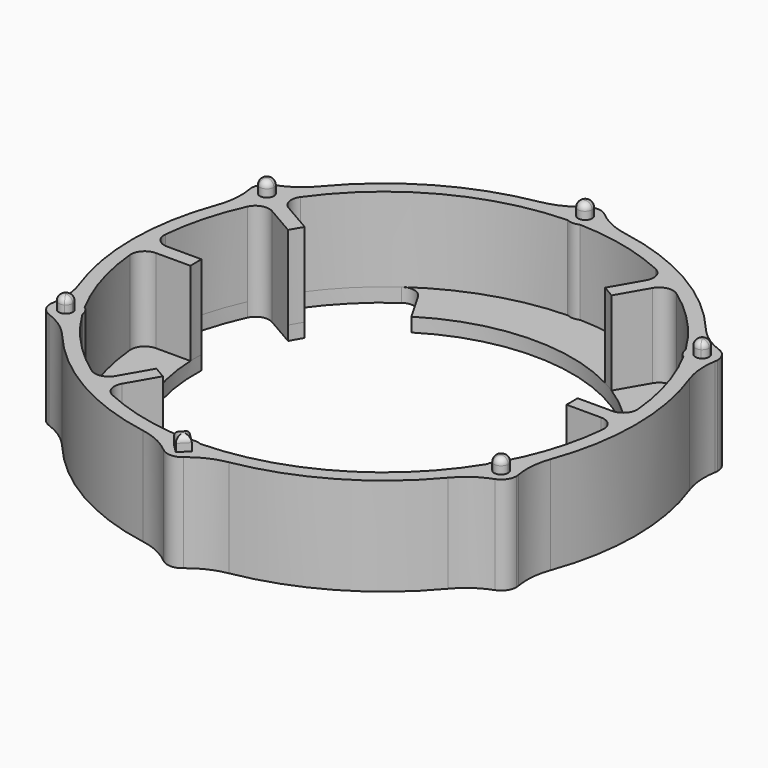
from build123d import *

# Parameters (mm, degrees)
F1_R         = 18
F1_R_2       = 17
F2_DEPTH     = 7
F3_DEPTH     = 7
F4_DEPTH     = 1
F6_DEPTH     = 7
F7_R         = 1
F8_R         = 5
F9_DEPTH     = 8
F10_R        = 0.44999
F11_DEPTH    = 1.8
F12_R        = 13.47
F13_DEPTH    = 1
F14_DEPTH    = 1
F15_T1_DEPTH = 1
F15_T3_DEPTH = 3.7395798703


# Not quite as in the source:
# - a fillet or chamfer that OpenCascade refuses, or shapes differently, is made with other operations: its cross-section is extruded or revolved along the edge and cut away or added
# - a fillet or chamfer is up to 0.001 mm smaller than in the source, because OpenCascade refuses the exact size


with BuildPart() as f2:
    # F1 (on Top) → F2 (new body)
    with BuildSketch(Plane.XY):
        Circle(F1_R)
        Circle(F1_R_2, mode=Mode.SUBTRACT)
    extrude(amount=F2_DEPTH)

    # F0 (on Top) → F3 (join)
    with BuildSketch(Plane.XY):
        with BuildLine():
            Line((-11.4073228059, 7.1633711619), (-14.4660626528, 8.9293354359))
            ThreePointArc((-14.4660626528, 8.9293354359), (-14.7224318643, 8.5), (-14.9660626528, 8.0633100321))
            Line((-14.9660626528, 8.0633100321), (-11.9073228059, 6.2973457581))
            ThreePointArc((-11.9073228059, 6.2973457581), (-11.665362189, 6.735), (-11.4073228059, 7.1633711619))
        make_face()
        with BuildLine():
            Line((7.1633711619, 11.4073228059), (8.9293354359, 14.4660626528))
            ThreePointArc((8.9293354359, 14.4660626528), (8.5, 14.7224318643), (8.0633100321, 14.9660626528))
            Line((8.0633100321, 14.9660626528), (6.2973457581, 11.9073228059))
            ThreePointArc((6.2973457581, 11.9073228059), (6.735, 11.665362189), (7.1633711619, 11.4073228059))
        make_face()
        with BuildLine():
            ThreePointArc((17, 0), (16.9981612676, 0.2500270431), (16.992645468, 0.5))
            Line((16.992645468, 0.5), (13.46071692, 0.5))
            ThreePointArc((13.46071692, 0.5), (13.46767903, 0.2500430841), (13.47, 0))
            ThreePointArc((13.47, 0), (13.46767903, -0.2500430841), (13.46071692, -0.5))
            Line((13.46071692, -0.5), (16.992645468, -0.5))
            ThreePointArc((16.992645468, -0.5), (16.9981612676, -0.2500270431), (17, 0))
        make_face()
        with BuildLine():
            ThreePointArc((-8.9293354359, -14.4660626528), (-8.5, -14.7224318643), (-8.0633100321, -14.9660626528))
            Line((-8.0633100321, -14.9660626528), (-6.2973457581, -11.9073228059))
            ThreePointArc((-6.2973457581, -11.9073228059), (-6.735, -11.665362189), (-7.1633711619, -11.4073228059))
            Line((-7.1633711619, -11.4073228059), (-8.9293354359, -14.4660626528))
        make_face()
        with BuildLine():
            Line((-13.46071692, 0.5), (-16.992645468, 0.5))
            ThreePointArc((-16.992645468, 0.5), (-17, 0), (-16.992645468, -0.5))
            Line((-16.992645468, -0.5), (-13.46071692, -0.5))
            ThreePointArc((-13.46071692, -0.5), (-13.47, 0), (-13.46071692, 0.5))
        make_face()
    extrude(amount=F3_DEPTH)

    # F1 (on Top) → F4 (join)
    with BuildSketch(Plane.XY):
        Circle(F1_R)
        Circle(F1_R_2, mode=Mode.SUBTRACT)
        Circle(F1_R_2)
    extrude(amount=F4_DEPTH)

    # F5 (on Top) → F6 (join)
    with BuildSketch(Plane.XY):
        with BuildLine():
            ThreePointArc((-14.4884572681, 9), (-14.6275367743, 9.5353800561), (-15.0096060035, 9.935377578))
            ThreePointArc((-15.0096060035, 9.935377578), (-15.1731450826, 9.6837837802), (-15.3324673166, 9.4294987133))
            ThreePointArc((-15.3324673166, 9.4294987133), (-15.153718855, 9.2469868663), (-15.0884572681, 9))
            ThreePointArc((-15.0884572681, 9), (-15.3354561915, 8.5687338928), (-15.832419089, 8.5635568422))
            ThreePointArc((-15.832419089, 8.5635568422), (-15.9729752997, 8.2984372068), (-16.1090923805, 8.0310113108))
            ThreePointArc((-16.1090923805, 8.0310113108), (-15.0239657375, 8.0558870238), (-14.4884572681, 9))
        make_face()
        with BuildLine():
            ThreePointArc((-15.3324673166, 9.4294987133), (-15.1731450826, 9.6837837802), (-15.0096060035, 9.935377578))
            ThreePointArc((-15.0096060035, 9.935377578), (-16.5410852123, 9.55), (-16.1090923805, 8.0310113108))
            ThreePointArc((-16.1090923805, 8.0310113108), (-15.9729752997, 8.2984372068), (-15.832419089, 8.5635568422))
            ThreePointArc((-15.832419089, 8.5635568422), (-16.02146997, 9.25), (-15.3324673166, 9.4294987133))
        make_face()
        with BuildLine():
            ThreePointArc((-1.099486377, 17.9663888889), (0, 16.9), (1.099486377, 17.9663888889))
            ThreePointArc((1.099486377, 17.9663888889), (0.7998302171, 17.982220987), (0.4999517724, 17.9930555556))
            ThreePointArc((0.4999517724, 17.9930555556), (0, 17.5), (-0.4999517724, 17.9930555556))
            ThreePointArc((-0.4999517724, 17.9930555556), (-0.7998302171, 17.982220987), (-1.099486377, 17.9663888889))
        make_face()
        with BuildLine():
            ThreePointArc((0.4999517724, 17.9930555556), (0.7998302171, 17.982220987), (1.099486377, 17.9663888889))
            ThreePointArc((1.099486377, 17.9663888889), (1.0998715868, 17.9831924823), (1.1, 18))
            ThreePointArc((1.1, 18), (-0.0168075177, 19.0998715868), (-1.099486377, 17.9663888889))
            ThreePointArc((-1.099486377, 17.9663888889), (-0.7998302171, 17.982220987), (-0.4999517724, 17.9930555556))
            ThreePointArc((-0.4999517724, 17.9930555556), (-0.003472306, 18.4999879429), (0.5, 18))
            ThreePointArc((0.5, 18), (0.4999879429, 17.996527694), (0.4999517724, 17.9930555556))
        make_face()
        with BuildLine():
            ThreePointArc((15.832419089, 8.5635568422), (15.9729752997, 8.2984372068), (16.1090923805, 8.0310113108))
            ThreePointArc((16.1090923805, 8.0310113108), (16.5325702443, 8.4355084694), (16.6884572681, 9))
            ThreePointArc((16.6884572681, 9), (16.1238373242, 9.9609204939), (15.0096060035, 9.935377578))
            ThreePointArc((15.0096060035, 9.935377578), (15.1731450826, 9.6837837802), (15.3324673166, 9.4294987133))
            ThreePointArc((15.3324673166, 9.4294987133), (15.8354441344, 9.4347384132), (16.0884572681, 9))
            ThreePointArc((16.0884572681, 9), (16.0197233753, 8.7469989234), (15.832419089, 8.5635568422))
        make_face()
        with BuildLine():
            ThreePointArc((15.0096060035, 9.935377578), (14.635829324, 8.45), (16.1090923805, 8.0310113108))
            ThreePointArc((16.1090923805, 8.0310113108), (15.9729752997, 8.2984372068), (15.832419089, 8.5635568422))
            ThreePointArc((15.832419089, 8.5635568422), (15.1554445662, 8.75), (15.3324673166, 9.4294987133))
            ThreePointArc((15.3324673166, 9.4294987133), (15.1731450826, 9.6837837802), (15.0096060035, 9.935377578))
        make_face()
        with BuildLine():
            ThreePointArc((-15.3324673166, -9.4294987133), (-15.1731450826, -9.6837837802), (-15.0096060035, -9.935377578))
            ThreePointArc((-15.0096060035, -9.935377578), (-14.6275367743, -9.5353800561), (-14.4884572681, -9))
            ThreePointArc((-14.4884572681, -9), (-15.0239657375, -8.0558870238), (-16.1090923805, -8.0310113108))
            ThreePointArc((-16.1090923805, -8.0310113108), (-15.9729752997, -8.2984372068), (-15.832419089, -8.5635568422))
            ThreePointArc((-15.832419089, -8.5635568422), (-15.3354561915, -8.5687338928), (-15.0884572681, -9))
            ThreePointArc((-15.0884572681, -9), (-15.153718855, -9.2469868663), (-15.3324673166, -9.4294987133))
        make_face()
        with BuildLine():
            ThreePointArc((-16.1090923805, -8.0310113108), (-16.5410852123, -9.55), (-15.0096060035, -9.935377578))
            ThreePointArc((-15.0096060035, -9.935377578), (-15.1731450826, -9.6837837802), (-15.3324673166, -9.4294987133))
            ThreePointArc((-15.3324673166, -9.4294987133), (-16.02146997, -9.25), (-15.832419089, -8.5635568422))
            ThreePointArc((-15.832419089, -8.5635568422), (-15.9729752997, -8.2984372068), (-16.1090923805, -8.0310113108))
        make_face()
        with BuildLine():
            ThreePointArc((0.6255239257, -17.9891278226), (0.8625800837, -17.9793202207), (1.099486377, -17.9663888889))
            ThreePointArc((1.099486377, -17.9663888889), (0, -16.9), (-1.099486377, -17.9663888889))
            ThreePointArc((-1.099486377, -17.9663888889), (-0.8625800837, -17.9793202207), (-0.6255239257, -17.9891278226))
            Line((-0.6255239257, -17.9891278226), (0, -17.3636038969))
            Line((0, -17.3636038969), (0.6255239257, -17.9891278226))
        make_face()
        with BuildLine():
            ThreePointArc((1.1, -18), (1.0998715868, -17.9831924823), (1.099486377, -17.9663888889))
            ThreePointArc((1.099486377, -17.9663888889), (0.8625800837, -17.9793202207), (0.6255239257, -17.9891278226))
            Line((0.6255239257, -17.9891278226), (0.6363961031, -18))
            Line((0.6363961031, -18), (0, -18.6363961031))
            Line((0, -18.6363961031), (-0.6363961031, -18))
            Line((-0.6363961031, -18), (-0.6255239257, -17.9891278226))
            ThreePointArc((-0.6255239257, -17.9891278226), (-0.8625800837, -17.9793202207), (-1.099486377, -17.9663888889))
            ThreePointArc((-1.099486377, -17.9663888889), (-0.0168075177, -19.0998715868), (1.1, -18))
        make_face()
        with BuildLine():
            ThreePointArc((16.6884572681, -9), (16.5325702443, -8.4355084694), (16.1090923805, -8.0310113108))
            ThreePointArc((16.1090923805, -8.0310113108), (15.9729752997, -8.2984372068), (15.832419089, -8.5635568422))
            ThreePointArc((15.832419089, -8.5635568422), (16.0197233753, -8.7469989234), (16.0884572681, -9))
            ThreePointArc((16.0884572681, -9), (15.8354441344, -9.4347384132), (15.3324673166, -9.4294987133))
            ThreePointArc((15.3324673166, -9.4294987133), (15.1731450826, -9.6837837802), (15.0096060035, -9.935377578))
            ThreePointArc((15.0096060035, -9.935377578), (16.1238373242, -9.9609204939), (16.6884572681, -9))
        make_face()
        with BuildLine():
            ThreePointArc((15.832419089, -8.5635568422), (15.9729752997, -8.2984372068), (16.1090923805, -8.0310113108))
            ThreePointArc((16.1090923805, -8.0310113108), (14.635829324, -8.45), (15.0096060035, -9.935377578))
            ThreePointArc((15.0096060035, -9.935377578), (15.1731450826, -9.6837837802), (15.3324673166, -9.4294987133))
            ThreePointArc((15.3324673166, -9.4294987133), (15.1554445662, -8.75), (15.832419089, -8.5635568422))
        make_face()
        with BuildLine():
            ThreePointArc((-15.0884572681, 9), (-15.153718855, 9.2469868663), (-15.3324673166, 9.4294987133))
            ThreePointArc((-15.3324673166, 9.4294987133), (-15.5884572681, 9), (-15.832419089, 8.5635568422))
            ThreePointArc((-15.832419089, 8.5635568422), (-15.3354561915, 8.5687338928), (-15.0884572681, 9))
        make_face()
        with BuildLine():
            ThreePointArc((-15.832419089, 8.5635568422), (-15.5884572681, 9), (-15.3324673166, 9.4294987133))
            ThreePointArc((-15.3324673166, 9.4294987133), (-16.02146997, 9.25), (-15.832419089, 8.5635568422))
        make_face()
        with BuildLine():
            ThreePointArc((-0.4999517724, 17.9930555556), (0, 18), (0.4999517724, 17.9930555556))
            ThreePointArc((0.4999517724, 17.9930555556), (0.4999879429, 17.996527694), (0.5, 18))
            ThreePointArc((0.5, 18), (-0.003472306, 18.4999879429), (-0.4999517724, 17.9930555556))
        make_face()
        with BuildLine():
            ThreePointArc((-0.4999517724, 17.9930555556), (0, 17.5), (0.4999517724, 17.9930555556))
            ThreePointArc((0.4999517724, 17.9930555556), (0, 18), (-0.4999517724, 17.9930555556))
        make_face()
        with BuildLine():
            ThreePointArc((15.3324673166, 9.4294987133), (15.5884572681, 9), (15.832419089, 8.5635568422))
            ThreePointArc((15.832419089, 8.5635568422), (16.0197233753, 8.7469989234), (16.0884572681, 9))
            ThreePointArc((16.0884572681, 9), (15.8354441344, 9.4347384132), (15.3324673166, 9.4294987133))
        make_face()
        with BuildLine():
            ThreePointArc((15.3324673166, 9.4294987133), (15.1554445662, 8.75), (15.832419089, 8.5635568422))
            ThreePointArc((15.832419089, 8.5635568422), (15.5884572681, 9), (15.3324673166, 9.4294987133))
        make_face()
        with BuildLine():
            ThreePointArc((16.0884572681, -9), (16.0197233753, -8.7469989234), (15.832419089, -8.5635568422))
            ThreePointArc((15.832419089, -8.5635568422), (15.5884572681, -9), (15.3324673166, -9.4294987133))
            ThreePointArc((15.3324673166, -9.4294987133), (15.8354441344, -9.4347384132), (16.0884572681, -9))
        make_face()
        with BuildLine():
            ThreePointArc((15.3324673166, -9.4294987133), (15.5884572681, -9), (15.832419089, -8.5635568422))
            ThreePointArc((15.832419089, -8.5635568422), (15.1554445662, -8.75), (15.3324673166, -9.4294987133))
        make_face()
        with BuildLine():
            Line((0.6363961031, -18), (0.6255239257, -17.9891278226))
            ThreePointArc((0.6255239257, -17.9891278226), (0, -18), (-0.6255239257, -17.9891278226))
            Line((-0.6255239257, -17.9891278226), (-0.6363961031, -18))
            Line((-0.6363961031, -18), (0, -18.6363961031))
            Line((0, -18.6363961031), (0.6363961031, -18))
        make_face()
        with BuildLine():
            ThreePointArc((-15.832419089, -8.5635568422), (-16.02146997, -9.25), (-15.3324673166, -9.4294987133))
            ThreePointArc((-15.3324673166, -9.4294987133), (-15.5884572681, -9), (-15.832419089, -8.5635568422))
        make_face()
        with BuildLine():
            ThreePointArc((-15.832419089, -8.5635568422), (-15.5884572681, -9), (-15.3324673166, -9.4294987133))
            ThreePointArc((-15.3324673166, -9.4294987133), (-15.153718855, -9.2469868663), (-15.0884572681, -9))
            ThreePointArc((-15.0884572681, -9), (-15.3354561915, -8.5687338928), (-15.832419089, -8.5635568422))
        make_face()
        with BuildLine():
            ThreePointArc((-0.6255239257, -17.9891278226), (0, -18), (0.6255239257, -17.9891278226))
            Line((0.6255239257, -17.9891278226), (0, -17.3636038969))
            Line((0, -17.3636038969), (-0.6255239257, -17.9891278226))
        make_face()
    extrude(amount=F6_DEPTH)

    # F7
    f7_edges = [f2.edges().sort_by_distance(p)[0] for p in [
        (-8.929335, -14.466063, 4),
        (-16.992645, 0.5, 4),
        (-14.466063, 8.929335, 4),
        (8.06331, 14.966063, 4),
        (16.992645, -0.5, 4),
        (-14.966063, 8.06331, 4),
        (-16.992645, -0.5, 4),
        (-8.06331, -14.966063, 4),
        (8.929335, 14.466063, 4),
        (16.992645, 0.5, 4),
    ]]
    fillet(f7_edges, radius=F7_R)

    # F8 (call 1 of 12: OpenCascade refuses the feature's edges together)
    f8_edges = [f2.edges().sort_by_distance(p)[0] for p in [
        (-16.109092, 8.031011, 3.5),
    ]]
    fillet(f8_edges, radius=F8_R)

    # F8#2 (call 2 of 12)
    f8_2_edges = [f2.edges().sort_by_distance(p)[0] for p in [
        (-15.009606, 9.935378, 3.5),
    ]]
    fillet(f8_2_edges, radius=F8_R)

    # F8#3 (call 3 of 12)
    f8_3_edges = [f2.edges().sort_by_distance(p)[0] for p in [
        (-1.099486, 17.966389, 3.5),
    ]]
    fillet(f8_3_edges, radius=F8_R)

    # F8#4 (call 4 of 12)
    f8_4_edges = [f2.edges().sort_by_distance(p)[0] for p in [
        (1.099486, 17.966389, 3.5),
    ]]
    fillet(f8_4_edges, radius=F8_R)

    # F8#5 (call 5 of 12)
    f8_5_edges = [f2.edges().sort_by_distance(p)[0] for p in [
        (-15.009606, -9.935378, 3.5),
    ]]
    fillet(f8_5_edges, radius=F8_R)

    # F8#6 (call 6 of 12)
    f8_6_edges = [f2.edges().sort_by_distance(p)[0] for p in [
        (-16.109092, -8.031011, 3.5),
    ]]
    fillet(f8_6_edges, radius=F8_R)

    # F8#7 (call 7 of 12)
    f8_7_edges = [f2.edges().sort_by_distance(p)[0] for p in [
        (1.099486, -17.966389, 3.5),
    ]]
    fillet(f8_7_edges, radius=F8_R)

    # F8#8 (call 8 of 12)
    f8_8_edges = [f2.edges().sort_by_distance(p)[0] for p in [
        (-1.099486, -17.966389, 3.5),
    ]]
    fillet(f8_8_edges, radius=F8_R)

    # F8#10 (call 9 of 12)
    f8_10_edges = [f2.edges().sort_by_distance(p)[0] for p in [
        (15.009606, -9.935378, 3.5),
    ]]
    fillet(f8_10_edges, radius=F8_R)

    # F8#11 (call 10 of 12)
    f8_11_edges = [f2.edges().sort_by_distance(p)[0] for p in [
        (16.109092, 8.031011, 3.5),
    ]]
    fillet(f8_11_edges, radius=F8_R)

    # F8#12 (call 11 of 12)
    f8_12_edges = [f2.edges().sort_by_distance(p)[0] for p in [
        (15.009606, 9.935378, 3.5),
    ]]
    fillet(f8_12_edges, radius=F8_R)

    # F8#9 (call 12 of 12)
    f8_9_edges = [f2.edges().sort_by_distance(p)[0] for p in [
        (16.109092, -8.031011, 3.5),
    ]]
    fillet(f8_9_edges, radius=F8_R)

    # F5 (on Top) → F9 (join)
    with BuildSketch(Plane.XY):
        with BuildLine():
            ThreePointArc((-15.832419089, 8.5635568422), (-15.5884572681, 9), (-15.3324673166, 9.4294987133))
            ThreePointArc((-15.3324673166, 9.4294987133), (-16.02146997, 9.25), (-15.832419089, 8.5635568422))
        make_face()
        with BuildLine():
            ThreePointArc((-15.0884572681, 9), (-15.153718855, 9.2469868663), (-15.3324673166, 9.4294987133))
            ThreePointArc((-15.3324673166, 9.4294987133), (-15.5884572681, 9), (-15.832419089, 8.5635568422))
            ThreePointArc((-15.832419089, 8.5635568422), (-15.3354561915, 8.5687338928), (-15.0884572681, 9))
        make_face()
        with BuildLine():
            ThreePointArc((-0.4999517724, 17.9930555556), (0, 18), (0.4999517724, 17.9930555556))
            ThreePointArc((0.4999517724, 17.9930555556), (0.4999879429, 17.996527694), (0.5, 18))
            ThreePointArc((0.5, 18), (-0.003472306, 18.4999879429), (-0.4999517724, 17.9930555556))
        make_face()
        with BuildLine():
            ThreePointArc((-0.4999517724, 17.9930555556), (0, 17.5), (0.4999517724, 17.9930555556))
            ThreePointArc((0.4999517724, 17.9930555556), (0, 18), (-0.4999517724, 17.9930555556))
        make_face()
        with BuildLine():
            ThreePointArc((15.3324673166, 9.4294987133), (15.1554445662, 8.75), (15.832419089, 8.5635568422))
            ThreePointArc((15.832419089, 8.5635568422), (15.5884572681, 9), (15.3324673166, 9.4294987133))
        make_face()
        with BuildLine():
            ThreePointArc((15.3324673166, 9.4294987133), (15.5884572681, 9), (15.832419089, 8.5635568422))
            ThreePointArc((15.832419089, 8.5635568422), (16.0197233753, 8.7469989234), (16.0884572681, 9))
            ThreePointArc((16.0884572681, 9), (15.8354441344, 9.4347384132), (15.3324673166, 9.4294987133))
        make_face()
        with BuildLine():
            ThreePointArc((15.3324673166, -9.4294987133), (15.5884572681, -9), (15.832419089, -8.5635568422))
            ThreePointArc((15.832419089, -8.5635568422), (15.1554445662, -8.75), (15.3324673166, -9.4294987133))
        make_face()
        with BuildLine():
            ThreePointArc((16.0884572681, -9), (16.0197233753, -8.7469989234), (15.832419089, -8.5635568422))
            ThreePointArc((15.832419089, -8.5635568422), (15.5884572681, -9), (15.3324673166, -9.4294987133))
            ThreePointArc((15.3324673166, -9.4294987133), (15.8354441344, -9.4347384132), (16.0884572681, -9))
        make_face()
        with BuildLine():
            Line((0.6363961031, -18), (0.6255239257, -17.9891278226))
            ThreePointArc((0.6255239257, -17.9891278226), (0, -18), (-0.6255239257, -17.9891278226))
            Line((-0.6255239257, -17.9891278226), (-0.6363961031, -18))
            Line((-0.6363961031, -18), (0, -18.6363961031))
            Line((0, -18.6363961031), (0.6363961031, -18))
        make_face()
        with BuildLine():
            ThreePointArc((-0.6255239257, -17.9891278226), (0, -18), (0.6255239257, -17.9891278226))
            Line((0.6255239257, -17.9891278226), (0, -17.3636038969))
            Line((0, -17.3636038969), (-0.6255239257, -17.9891278226))
        make_face()
        with BuildLine():
            ThreePointArc((-15.832419089, -8.5635568422), (-16.02146997, -9.25), (-15.3324673166, -9.4294987133))
            ThreePointArc((-15.3324673166, -9.4294987133), (-15.5884572681, -9), (-15.832419089, -8.5635568422))
        make_face()
        with BuildLine():
            ThreePointArc((-15.832419089, -8.5635568422), (-15.5884572681, -9), (-15.3324673166, -9.4294987133))
            ThreePointArc((-15.3324673166, -9.4294987133), (-15.153718855, -9.2469868663), (-15.0884572681, -9))
            ThreePointArc((-15.0884572681, -9), (-15.3354561915, -8.5687338928), (-15.832419089, -8.5635568422))
        make_face()
    extrude(amount=F9_DEPTH)

    # F10 (radius 0.45 in the source; OpenCascade refuses exactly that, so slightly less here)
    f10_edges = [f2.edges().sort_by_distance(p)[0] for p in [
        (-15.844447, -8.570501, 8),
        (-15.344495, 9.436443, 8),
        (0.499952, 18.006944, 8),
        (15.344495, 9.436443, 8),
        (15.844447, -8.570501, 8),
        (0.318198, -17.681802, 8),
        (-0.318198, -18.318198, 8),
        (0.318198, -18.318198, 8),
        (-0.318198, -17.681802, 8),
    ]]
    fillet(f10_edges, radius=F10_R)

    # F5 (on Top) → F11 (cut)
    with BuildSketch(Plane.XY):
        with BuildLine():
            ThreePointArc((-15.832419089, -8.5635568422), (-16.02146997, -9.25), (-15.3324673166, -9.4294987133))
            ThreePointArc((-15.3324673166, -9.4294987133), (-15.5884572681, -9), (-15.832419089, -8.5635568422))
        make_face()
        with BuildLine():
            ThreePointArc((-15.832419089, -8.5635568422), (-15.5884572681, -9), (-15.3324673166, -9.4294987133))
            ThreePointArc((-15.3324673166, -9.4294987133), (-15.153718855, -9.2469868663), (-15.0884572681, -9))
            ThreePointArc((-15.0884572681, -9), (-15.3354561915, -8.5687338928), (-15.832419089, -8.5635568422))
        make_face()
        with BuildLine():
            Line((0.6363961031, -18), (0.6255239257, -17.9891278226))
            ThreePointArc((0.6255239257, -17.9891278226), (0, -18), (-0.6255239257, -17.9891278226))
            Line((-0.6255239257, -17.9891278226), (-0.6363961031, -18))
            Line((-0.6363961031, -18), (0, -18.6363961031))
            Line((0, -18.6363961031), (0.6363961031, -18))
        make_face()
        with BuildLine():
            ThreePointArc((-0.6255239257, -17.9891278226), (0, -18), (0.6255239257, -17.9891278226))
            Line((0.6255239257, -17.9891278226), (0, -17.3636038969))
            Line((0, -17.3636038969), (-0.6255239257, -17.9891278226))
        make_face()
        with BuildLine():
            ThreePointArc((15.3324673166, -9.4294987133), (15.5884572681, -9), (15.832419089, -8.5635568422))
            ThreePointArc((15.832419089, -8.5635568422), (15.1554445662, -8.75), (15.3324673166, -9.4294987133))
        make_face()
        with BuildLine():
            ThreePointArc((16.0884572681, -9), (16.0197233753, -8.7469989234), (15.832419089, -8.5635568422))
            ThreePointArc((15.832419089, -8.5635568422), (15.5884572681, -9), (15.3324673166, -9.4294987133))
            ThreePointArc((15.3324673166, -9.4294987133), (15.8354441344, -9.4347384132), (16.0884572681, -9))
        make_face()
        with BuildLine():
            ThreePointArc((15.3324673166, 9.4294987133), (15.1554445662, 8.75), (15.832419089, 8.5635568422))
            ThreePointArc((15.832419089, 8.5635568422), (15.5884572681, 9), (15.3324673166, 9.4294987133))
        make_face()
        with BuildLine():
            ThreePointArc((15.3324673166, 9.4294987133), (15.5884572681, 9), (15.832419089, 8.5635568422))
            ThreePointArc((15.832419089, 8.5635568422), (16.0197233753, 8.7469989234), (16.0884572681, 9))
            ThreePointArc((16.0884572681, 9), (15.8354441344, 9.4347384132), (15.3324673166, 9.4294987133))
        make_face()
        with BuildLine():
            ThreePointArc((-0.4999517724, 17.9930555556), (0, 17.5), (0.4999517724, 17.9930555556))
            ThreePointArc((0.4999517724, 17.9930555556), (0, 18), (-0.4999517724, 17.9930555556))
        make_face()
        with BuildLine():
            ThreePointArc((-0.4999517724, 17.9930555556), (0, 18), (0.4999517724, 17.9930555556))
            ThreePointArc((0.4999517724, 17.9930555556), (0.4999879429, 17.996527694), (0.5, 18))
            ThreePointArc((0.5, 18), (-0.003472306, 18.4999879429), (-0.4999517724, 17.9930555556))
        make_face()
        with BuildLine():
            ThreePointArc((-15.832419089, 8.5635568422), (-15.5884572681, 9), (-15.3324673166, 9.4294987133))
            ThreePointArc((-15.3324673166, 9.4294987133), (-16.02146997, 9.25), (-15.832419089, 8.5635568422))
        make_face()
        with BuildLine():
            ThreePointArc((-15.0884572681, 9), (-15.153718855, 9.2469868663), (-15.3324673166, 9.4294987133))
            ThreePointArc((-15.3324673166, 9.4294987133), (-15.5884572681, 9), (-15.832419089, 8.5635568422))
            ThreePointArc((-15.832419089, 8.5635568422), (-15.3354561915, 8.5687338928), (-15.0884572681, 9))
        make_face()
    extrude(amount=F11_DEPTH, mode=Mode.SUBTRACT)

    # F12 (on Top) → F13 (cut)
    with BuildSketch(Plane.XY):
        Circle(F12_R)
    extrude(amount=F13_DEPTH, mode=Mode.SUBTRACT)

    # F0 (on Top) → F14 (cut)
    with BuildSketch(Plane.XY):
        with BuildLine():
            Line((13.46071692, 0.5), (16.992645468, 0.5))
            ThreePointArc((16.992645468, 0.5), (16.4207390469, 4.3999237667), (14.9660626528, 8.0633100321))
            Line((14.9660626528, 8.0633100321), (11.9073228059, 6.2973457581))
            ThreePointArc((11.9073228059, 6.2973457581), (13.0110208801, 3.4862925375), (13.46071692, 0.5))
        make_face()
        with BuildLine():
            Line((-7.1633711619, 11.4073228059), (-8.9293354359, 14.4660626528))
            ThreePointArc((-8.9293354359, 14.4660626528), (-12.0208152802, 12.0208152802), (-14.4660626528, 8.9293354359))
            Line((-14.4660626528, 8.9293354359), (-11.4073228059, 7.1633711619))
            ThreePointArc((-11.4073228059, 7.1633711619), (-9.5247283426, 9.5247283426), (-7.1633711619, 11.4073228059))
        make_face()
        with BuildLine():
            Line((-11.9073228059, 6.2973457581), (-14.9660626528, 8.0633100321))
            ThreePointArc((-14.9660626528, 8.0633100321), (-16.4207390469, 4.3999237667), (-16.992645468, 0.5))
            Line((-16.992645468, 0.5), (-13.46071692, 0.5))
            ThreePointArc((-13.46071692, 0.5), (-13.0110208801, 3.4862925375), (-11.9073228059, 6.2973457581))
        make_face()
    extrude(amount=F14_DEPTH, mode=Mode.SUBTRACT)

    # F15: fillet of radius 1 on 6 edges, made by hand

    # F15_s2 → F15_t1 (join)
    with BuildSketch(Plane.XY):
        with BuildLine():
            ThreePointArc((-8.3977788629, 13.5453796613), (-9.0505980623, 14.0223868846), (-9.8427920334, 13.8607158902))
            ThreePointArc((-9.8427920334, 13.8607158902), (-9.3909426367, 14.1707514407), (-8.9293354359, 14.4660626528))
            Line((-8.9293354359, 14.4660626528), (-8.3977788629, 13.5453796613))
        make_face()
        with BuildLine():
            ThreePointArc((14.0453796613, 7.5317534591), (14.8492412838, 7.6184442326), (15.4544658902, 7.0823360588))
            ThreePointArc((15.4544658902, 7.0823360588), (15.2181706092, 7.57675942), (14.9660626528, 8.0633100321))
            Line((14.9660626528, 8.0633100321), (14.0453796613, 7.5317534591))
        make_face()
    extrude(amount=F15_T1_DEPTH)

    # F15_s4 → F15_t3 (join)
    with BuildSketch(Plane.XY):
        with BuildLine():
            ThreePointArc((-14.0453796613, 7.5317534591), (-14.8492412838, 7.6184442326), (-15.4544658902, 7.0823360588))
            ThreePointArc((-15.4544658902, 7.0823360588), (-15.2181706092, 7.57675942), (-14.9660626528, 8.0633100321))
            Line((-14.9660626528, 8.0633100321), (-14.0453796613, 7.5317534591))
        make_face()
        with BuildLine():
            ThreePointArc((-16.9251280922, 1.59375), (-16.669042295, 0.8268543991), (-15.9295323221, 0.5))
            Line((-15.9295323221, 0.5), (-16.992645468, 0.5))
            ThreePointArc((-16.992645468, 0.5), (-16.9677020567, 1.0474191685), (-16.9251280922, 1.59375))
        make_face()
        with BuildLine():
            ThreePointArc((16.9251280922, 1.59375), (16.669042295, 0.8268543991), (15.9295323221, 0.5))
            Line((15.9295323221, 0.5), (16.992645468, 0.5))
            ThreePointArc((16.992645468, 0.5), (16.9677020567, 1.0474191685), (16.9251280922, 1.59375))
        make_face()
        with BuildLine():
            ThreePointArc((-13.5453796613, 8.3977788629), (-14.0223868846, 9.0505980623), (-13.8607158902, 9.8427920334))
            ThreePointArc((-13.8607158902, 9.8427920334), (-14.1707514407, 9.3909426367), (-14.4660626528, 8.9293354359))
            Line((-14.4660626528, 8.9293354359), (-13.5453796613, 8.3977788629))
        make_face()
    extrude(amount=F15_T3_DEPTH)


solid = f2.part
